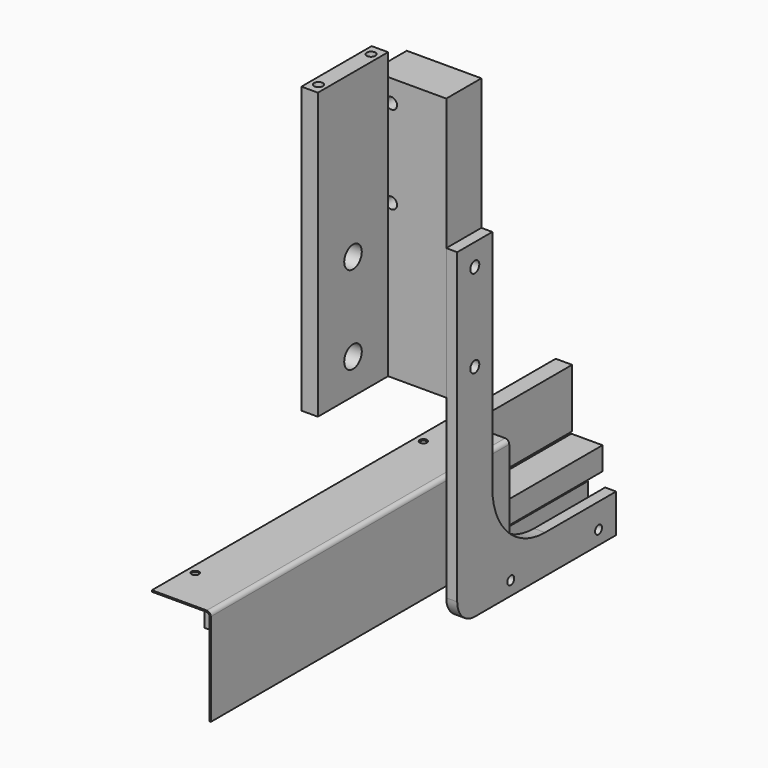
from build123d import *

# Parameters (mm, degrees)
F0_W      = 43.18
F0_H      = 152.4
F1_DEPTH  = 25.4
F2_D      = 6.5278
F3_W      = 50.8
F3_H      = 165.1
F4_DEPTH  = 9.525
F5_D      = 12.7
F7_D      = 5.1054
F7_DEPTH  = 12.7
F7_TIP    = 1.5338169022
F8_W      = 9.525
F8_H      = 33.8836
F9_DEPTH  = 127
F11_W     = 18.0086
F11_H     = 96
F12_DEPTH = 13.335
F14_D     = 3.3
F14_DEPTH = 10.16
F14_TIP   = 0.9914200214
F15_W     = 18.0086
F15_H     = 84.455
F15_R     = 1.65
F15_H_2   = 4.445
F15_W_2   = 9.9822
F15_H_3   = 88.9
F16_DEPTH = 19.05
F17_DEPTH = 9.525
F18_D     = 4.4
F20_D     = 4.0386
F20_DEPTH = 12.7
F20_TIP   = 1.213317848
F22_D     = 5.4102
F22_DEPTH = 13.0401785714
F22_TIP   = 1.6253880605
F23_W     = 25.4
F23_H     = 76.2
F23_R     = 2.7051
F23_W_2   = 88.9
F23_H_2   = 9.525
F24_DEPTH = 6.35
F26_D     = 6.5278
F27_D     = 4.9784
F28_R     = 12.7
F31_DEPTH = 215.9
F33_D     = 4.318


with BuildPart() as f1:
    # F0 (on Front) → F1 (new body)
    with BuildSketch(Plane.XZ):
        with Locations((21.59, 76.2)):
            Rectangle(F0_W, F0_H)
    extrude(amount=-F1_DEPTH)

    # F2 (through all)
    with Locations(Plane.XZ):
        with Locations((11.43, 139.7), (11.43, 88.9)):
            Hole(F2_D / 2)

    # F22
    with Locations(Plane.YZ.offset(43.18)):
        with Locations((12.7, 63.5), (12.7, 12.7)):
            Hole(F22_D / 2, depth=F22_DEPTH)
            with Locations((0, 0, -(F22_DEPTH + F22_TIP / 2))):  # 118° drill point
                Cone(0, F22_D / 2, F22_TIP, mode=Mode.SUBTRACT)


with BuildPart() as f4:
    # F3 (on Right) → F4 (new body)
    with BuildSketch(Plane.YZ):
        with Locations((-25.4, 82.55)):
            Rectangle(F3_W, F3_H)
    extrude(amount=F4_DEPTH)

    # F5 (through all)
    with Locations(Plane(origin=(0, 0, 0), x_dir=(0, 1, 0), z_dir=(-1, 0, 0))):
        with Locations((-25.4, -71.12), (-25.4, -20.32)):
            Hole(F5_D / 2)

    # F7
    with Locations(Plane.XY.offset(165.1)):
        with Locations((4.7625, -6.35), (4.7625, -44.45)):
            Hole(F7_D / 2, depth=F7_DEPTH)
            with Locations((0, 0, -(F7_DEPTH + F7_TIP / 2))):  # 118° drill point
                Cone(0, F7_D / 2, F7_TIP, mode=Mode.SUBTRACT)


with BuildPart() as f9:
    # F8 (on Front) → F9 (new body, symmetric)
    with BuildSketch(Plane.XZ):
        with Locations((9.6647, -61.1632)):
            Rectangle(F8_W, F8_H)
    extrude(amount=F9_DEPTH, both=True)


with BuildPart() as f12:
    # F11 (on offset) → F12 (new body)
    with BuildSketch(Plane(origin=(0, 0, -79.121), x_dir=(1, 0, 0), z_dir=(0, 0, -1))):
        with Locations((23.4315, -78.48)):
            Rectangle(F11_W, F11_H)
    extrude(amount=F12_DEPTH)

    # F14
    with Locations(Plane(origin=(0, 0, -92.456), x_dir=(1, 0, 0), z_dir=(0, 0, -1))):
        with Locations((29.4358, -33.4772), (17.4358, -107.4772)):
            Hole(F14_D / 2, depth=F14_DEPTH)
            with Locations((0, 0, -(F14_DEPTH + F14_TIP / 2))):  # 118° drill point
                Cone(0, F14_D / 2, F14_TIP, mode=Mode.SUBTRACT)


with BuildPart() as f16:
    # F15 (on face) → F16 (new body)
    with BuildSketch(Plane(origin=(0, 0, -92.456), x_dir=(1, 0, 0), z_dir=(0, 0, -1))):
        with Locations((23.4315, -72.7075)):
            Rectangle(F15_W, F15_H)
        with Locations((17.4358, -107.4772)):
            Circle(F15_R, mode=Mode.SUBTRACT)
        with Locations((29.4358, -33.4772)):
            Circle(F15_R, mode=Mode.SUBTRACT)
        with Locations((23.4315, -28.2575)):
            Rectangle(F15_W, F15_H_2)
        with Locations((38.1889, -70.485)):
            Rectangle(F15_W_2, F15_H_3)
        Polygon((14.4272, -30.48), (14.4272, -26.035), (13.6652, -26.035), (13.6652, -114.935), (14.4272, -114.935), align=None)
        Polygon((33.1978, -26.035), (32.4358, -26.035), (32.4358, -30.48), (32.4358, -114.935), (33.1978, -114.935), align=None)
    extrude(amount=F16_DEPTH)

    # F15 (on face) → F17 (cut)
    with BuildSketch(Plane(origin=(0, 0, -92.456), x_dir=(1, 0, 0), z_dir=(0, 0, -1))):
        with Locations((38.1889, -70.485)):
            Rectangle(F15_W_2, F15_H_3)
    extrude(amount=F17_DEPTH, mode=Mode.SUBTRACT)

    # F18 (through all)
    with Locations(Plane.XY.offset(-92.456)):
        with Locations((29.4358, 33.4772), (17.4358, 107.4772)):
            Hole(F18_D / 2)

    # F20
    with Locations(Plane.YZ.offset(43.18)):
        with Locations((38.735, -106.7435), (102.235, -106.7435)):
            Hole(F20_D / 2, depth=F20_DEPTH)
            with Locations((0, 0, -(F20_DEPTH + F20_TIP / 2))):  # 118° drill point
                Cone(0, F20_D / 2, F20_TIP, mode=Mode.SUBTRACT)


with BuildPart() as f24:
    # F23 (on face) → F24 (new body)
    with BuildSketch(Plane.YZ.offset(43.18)):
        with Locations((12.7, 38.1)):
            Rectangle(F23_W, F23_H)
        with Locations((12.7, 12.7)):
            Circle(F23_R, mode=Mode.SUBTRACT)
        with Locations((12.7, 63.5)):
            Circle(F23_R, mode=Mode.SUBTRACT)
        Polygon((26.035, -111.506), (26.035, -101.981), (25.4, -101.981), (25.4, -92.456), (25.4, -54.3559999772), (25.4, 0), (0, 0), (0, -111.506), align=None)
        Polygon((26.035, -101.981), (114.935, -101.981), (114.935, -92.456), (63.5, -92.456), (25.4, -92.456), (25.4, -101.981), align=None)
        with Locations((70.485, -106.7435)):
            Rectangle(F23_W_2, F23_H_2)
        with BuildLine():
            Line((25.4, -92.456), (63.5, -92.456))
            ThreePointArc((63.5, -92.456), (36.5592316287, -81.2967683551), (25.4, -54.3559999772))
            Line((25.4, -54.3559999772), (25.4, -92.456))
        make_face()
        Polygon((114.935, -114.681), (114.935, -111.506), (26.035, -111.506), (0, -111.506), (0, -114.681), align=None)
    extrude(amount=F24_DEPTH)

    # F26 (through all)
    with Locations(Plane.YZ.offset(49.53)):
        with Locations((12.7, 63.5), (12.7, 12.7)):
            Hole(F26_D / 2)

    # F27 (through all)
    with Locations(Plane.YZ.offset(49.53)):
        with Locations((38.735, -106.7435), (102.235, -106.7435)):
            Hole(F27_D / 2)

    # F28
    f28_edges = [f24.edges().sort_by_distance(p)[0] for p in [
        (46.355, 0, -114.681),
    ]]
    fillet(f28_edges, radius=F28_R)


with BuildPart() as f31:
    # F30 (on offset) → F31 (new body)
    with BuildSketch(Plane.XZ.offset(-50.8)):
        with BuildLine():
            Line((4.9022, -43.4086), (4.9022, -44.2214))
            Line((4.9022, -44.2214), (14.4272, -44.2214))
            Line((14.4272, -44.2214), (36.6141, -44.2214))
            ThreePointArc((36.6141, -44.2214), (37.727651759, -44.682648241), (38.1889, -45.7962))
            Line((38.1889, -45.7962), (38.1889, -99.441))
            Line((38.1889, -99.441), (39.0017, -99.441))
            Line((39.0017, -99.441), (39.0017, -45.7962))
            ThreePointArc((39.0017, -45.7962), (38.3023881508, -44.1079118492), (36.6141, -43.4086))
            Line((36.6141, -43.4086), (4.9022, -43.4086))
        make_face()
    extrude(amount=F31_DEPTH)

    # F33 (through all)
    with Locations(Plane.XY.offset(-43.4086)):
        with Locations((9.6647, -139.7), (9.6647, 25.4)):
            Hole(F33_D / 2)


solid = Compound([f1.part, f4.part, f9.part, f12.part, f16.part, f24.part, f31.part])
